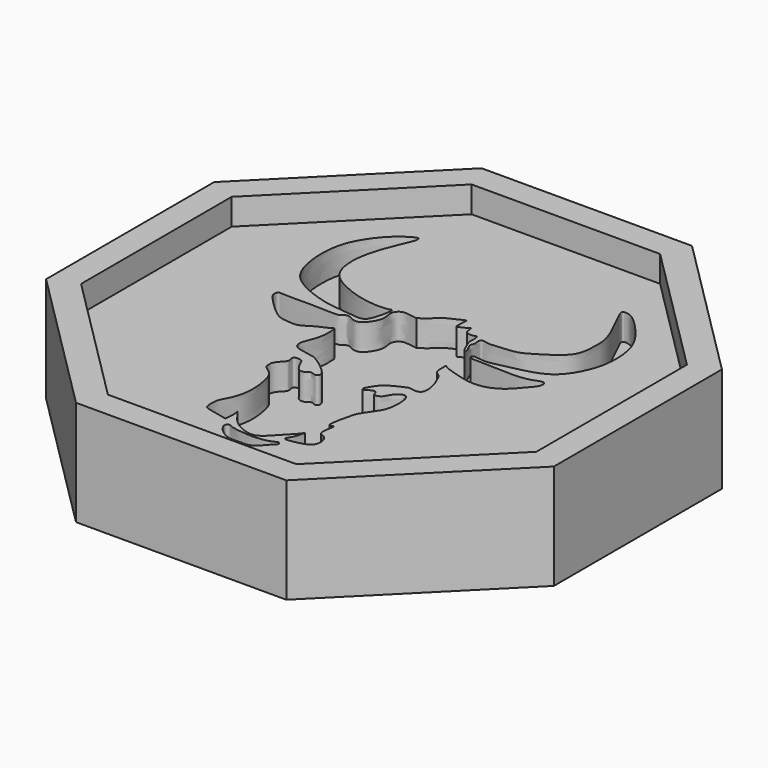
from build123d import *

# Parameters (mm, degrees)
F1_DEPTH = 25.4
F3_DEPTH = 6.35
F5_DEPTH = 6.35


with BuildPart() as f1:
    # F0 (on Top) → F1 (new body)
    with BuildSketch(Plane.XY):
        Polygon((-61.3372846899, 25.3607087968), (-61.3047391097, -25.4392807779), (-25.3607087968, -61.3372846899), (25.4392807779, -61.3047391097), (61.3372846899, -25.3607087968), (61.3047391097, 25.4392807779), (25.3607087968, 61.3372846899), (-25.4392807779, 61.3047391097), align=None)
    extrude(amount=F1_DEPTH)

    # F2 (on face) → F3 (cut)
    with BuildSketch(Plane.XY.offset(25.4)):
        Polygon((-54.9856008905, 22.734521413), (-54.9564255154, -22.8049569991), (-22.734521413, -54.9856008905), (22.8049569991, -54.9564255154), (54.9856008905, -22.734521413), (54.9564255154, 22.8049569991), (22.734521413, 54.9856008905), (-22.8049569991, 54.9564255154), align=None)
    extrude(amount=-F3_DEPTH, mode=Mode.SUBTRACT)

    # F4 (on face) → F5 (cut)
    with BuildSketch(Plane.XY.offset(19.05)):
        with BuildLine():
            add(Edge.make_bspline(
                [(-9.4282692298, -9.2326691374), (-8.4840850857, -9.8260777562), (-6.6516469636, -10.9777435428), (-4.395465984, -13.058877404), (-3.9906127923, -14.1891294159), (-4.8528640078, -15.0271217271), (-6.0855293908, -14.0647696181), (-6.8361021294, -15.0831488918), (-8.4800836888, -15.3844987998), (-9.4607258976, -13.8382234216), (-10.1783295199, -12.39132644), (-10.530585818, -11.4926907531), (-12.7551665659, -11.3984729667), (-12.4444668271, -12.6798354478), (-12.2593299659, -13.6545652797), (-13.6051622467, -14.7620446933), (-14.3409348224, -16.0220239486), (-14.321922051, -16.7704078365), (-14.3138650061, -17.9202545143), (-13.1186034777, -18.6564307431), (-11.4302528187, -20.0472476584), (-10.6225997404, -23.450310294), (-10.1147680829, -28.2741892714), (-11.7415790253, -32.6431531794), (-12.9174382916, -34.1649309464), (-12.9299587644, -37.178912773), (-12.4084055803, -38.2180544166), (-8.2145131464, -38.8077069126), (-6.8308559522, -39.4327185107), (-6.875484581, -38.16030542), (-6.6653450214, -36.0611878603), (-7.371128777, -34.9869994652), (-6.2460552937, -36.5408514888), (-4.4390102983, -39.0530569173), (-1.5015671125, -40.8477543068), (1.7071115917, -41.5564539503), (4.0576467306, -39.4557372162), (6.3424814353, -36.8930641139), (8.1590712868, -35.071811946), (8.5316472223, -34.1183133667), (8.2345836672, -35.2844855117), (7.8610398012, -37.1981099423), (6.2839273245, -38.9874526439), (9.266326691, -38.6346600876), (12.189835357, -37.8890680945), (13.4675883573, -36.1487373368), (12.7198460699, -33.0918695437), (9.930596948, -33.0395399652), (11.7099019289, -28.1494867023), (9.3191604838, -30.1136369501), (10.7720113651, -24.0356712037), (11.150243095, -22.091243294), (13.5772865075, -18.9251935606), (14.8003233954, -16.6011904572), (14.9201164538, -12.1791536076), (13.9622562681, -10.6026640562), (12.7803035011, -10.6938590154), (11.4362744481, -11.9801209333), (10.9312367978, -13.1215024658), (10.2453634757, -14.0686647647), (8.6352191248, -14.3879407439), (8.7073308617, -12.9044764652), (7.5209627677, -12.8396326003), (6.5256616405, -13.580406599), (6.0869976466, -13.9772738505), (5.4570005301, -13.5396377785), (6.3303917881, -11.9377003518), (7.7098741158, -9.8249117821), (11.0587187123, -8.2707570297), (12.4591243746, -7.6294322877), (13.4778087168, -8.1067590986), (15.9277607605, -7.9424041277), (15.2556568662, -3.8663568868), (14.4862990975, -2.3485813704), (13.7665382129, -0.3592892165), (12.2046730698, 0.3939785277), (12.0582121105, 1.6236098482), (12.0255761857, 3.9516208247), (12.4450103136, 3.1027423912), (16.5110699597, 1.8249579504), (21.078106057, 0.7115795625), (26.0638495162, 2.1812531443), (29.2230087502, 5.7843129757), (31.2737116624, 8.2182389542), (31.2278889418, 9.721207294), (30.0857203595, 9.9724642069), (28.472510997, 9.0185412307), (24.5513264234, 8.481216416), (19.6181854574, 8.7905574192), (16.196127468, 8.8653123167), (13.3446161645, 8.723991591), (13.4927937008, 10.2286844933), (16.4508103427, 9.2297816698), (21.1013365186, 10.502293822), (25.9735893436, 11.4472493706), (31.1878588966, 13.4941405465), (34.4638101564, 19.3145293919), (35.6394736154, 24.2110537108), (35.275960363, 31.6512720663), (31.1650423262, 37.2520467873), (28.0533420692, 40.3273925181), (26.4296452657, 41.485700122), (25.4190416812, 41.7070187418), (23.9748134483, 41.8669669932), (24.8551004672, 39.5530018645), (26.5847000727, 36.3840778799), (29.2164222614, 30.8323567036), (28.9476077056, 27.0951272934), (28.9521176027, 21.9651272091), (22.6263582287, 18.0817154192), (19.2763516356, 16.019175046), (15.6410149746, 16.0264947024), (12.6622540075, 15.4454248136), (11.1029074367, 16.2069281425), (10.3960461713, 15.3750494473), (10.8691535509, 13.7673825709), (10.1396442285, 13.0680734148), (11.0848560208, 11.6307606922), (11.6267048162, 9.8553781089), (10.3928447984, 11.2233156131), (9.7992288744, 13.040687065), (9.2598412935, 14.0477513552), (9.579696114, 15.9380770854), (9.0964793415, 16.8614094225), (8.4893205371, 16.2800428745), (6.8331120922, 16.4974540301), (6.4618248238, 16.8524107039), (6.1792797507, 19.1298816215), (5.9113327868, 18.1703634489), (4.4194509507, 17.7211838272), (3.4659487949, 16.9830424479), (3.5619819446, 18.4217518194), (3.5278446131, 19.5784882166), (3.7709848691, 20.6735203119), (2.3441332322, 19.9031610038), (-0.9966306201, 18.4935375741), (-2.3579134542, 16.6290500898), (-3.7437918395, 15.7644089715), (-4.4414699078, 15.3291318566)],
                knots=[0, 0, 0, 0, 0.0093887284, 0.0182213014, 0.0233131476, 0.0280114315, 0.0336124529, 0.0388132789, 0.0448508987, 0.0514661867, 0.0579869925, 0.0628125121, 0.0693776173, 0.0742962539, 0.0792086391, 0.0857519788, 0.0918428882, 0.096206218, 0.1013259694, 0.1071197189, 0.1144428534, 0.1237972835, 0.1352105935, 0.1459420833, 0.1531121172, 0.1615423232, 0.166725975, 0.1771658341, 0.1826563447, 0.1875106221, 0.1953019551, 0.1993991365, 0.2049196268, 0.2142540612, 0.2237371342, 0.2325054811, 0.2411782885, 0.2508781783, 0.2591627147, 0.2628089063, 0.2671087438, 0.2748303973, 0.2810510059, 0.288327223, 0.2974990844, 0.3045293751, 0.3127628534, 0.3198779695, 0.3291877075, 0.3339090751, 0.344899217, 0.3532071168, 0.3628568316, 0.371425535, 0.3819640039, 0.3883300936, 0.3932867711, 0.400116702, 0.405861066, 0.4113515785, 0.4169281938, 0.4220877311, 0.4269420071, 0.4326863712, 0.4363325684, 0.4397829616, 0.4461115588, 0.4544648842, 0.4642024659, 0.4702647327, 0.475518763, 0.4822836579, 0.4917234199, 0.4988296333, 0.5059693952, 0.5122407232, 0.5181217541, 0.5250173913, 0.5279604155, 0.5382313342, 0.5496481242, 0.5608846845, 0.5720957385, 0.5810687061, 0.5864740039, 0.5912025392, 0.597959558, 0.6080841791, 0.6195106459, 0.6293471359, 0.6371175574, 0.6412359933, 0.6492714977, 0.6606297825, 0.672079886, 0.6838871859, 0.6966594462, 0.7081745795, 0.7217890209, 0.7352308346, 0.7458378514, 0.752717581, 0.7579895334, 0.7629390765, 0.7696434146, 0.7798200645, 0.7922806096, 0.8021612881, 0.8130937866, 0.8265476592, 0.8367431308, 0.8462814452, 0.8551661805, 0.8613306134, 0.8658218009, 0.8721503975, 0.8766689416, 0.8833473635, 0.8888875665, 0.8942092607, 0.9015411068, 0.9070011411, 0.9140060991, 0.9183725406, 0.9224140492, 0.928747576, 0.932690837, 0.9394067292, 0.9425824756, 0.9492085016, 0.9537759532, 0.9588705435, 0.9648854784, 0.9691373246, 0.9744837396, 0.9843635518, 0.9921283086, 1, 1, 1, 1], degree=3))
            add(Edge.make_bspline(
                [(-4.4414699078, 15.3291318566), (-4.9068967225, 15.3806827308), (-5.9349556814, 15.4945509834), (-8.2732521375, 15.9847129393), (-9.7667880134, 14.1101988204), (-9.168903392, 12.2312839638), (-9.2484442212, 10.9020733102), (-9.7414335487, 9.5674071396), (-11.3511745418, 7.1567049444), (-13.3918709559, 7.1479473791), (-14.7050111685, 8.1215683651), (-15.5706019088, 7.9667355563), (-16.4311261821, 7.4484853366), (-16.6547257887, 6.9135346109), (-23.4598936578, 7.3918112186), (-29.3448714402, 7.1065466932), (-30.8844644754, 7.3670952023), (-31.5182667154, 7.3409536777), (-31.6997293932, 6.0030194205), (-30.7753763437, 4.6887419911), (-28.3533346738, 2.2006722005), (-24.863507439, -0.8319883365), (-22.4599240989, -0.7963354442), (-20.0140560821, -1.2610430772), (-17.5149487875, 0.8612721058), (-14.8122648285, 1.7088528475), (-14.3728875457, 2.3916052687), (-13.6860658167, 2.380095861), (-13.7189647119, 1.1992723358), (-13.4716632298, -1.5444326183), (-14.9295629485, -5.0303479787), (-15.3564223079, -6.3035501228), (-14.9174930287, -8.246461194), (-12.1365329972, -8.6339063958), (-10.3490742469, -9.0290908364), (-9.4282692298, -9.2326691374)],
                knots=[0, 0, 0, 0, 0.0267259922, 0.0590337618, 0.089461151, 0.1191102068, 0.1435366022, 0.1695820738, 0.2054113012, 0.2347455632, 0.26152597, 0.2813534837, 0.3022021384, 0.3158535767, 0.3709693963, 0.4262535041, 0.4514743551, 0.4660512479, 0.4886049281, 0.5155466217, 0.5566192303, 0.6029135136, 0.6357538083, 0.6683461724, 0.707524857, 0.7435858948, 0.7618014862, 0.7761487209, 0.797006954, 0.8338980252, 0.8758818035, 0.9011714843, 0.9284460361, 0.9631391499, 1, 1, 1, 1], degree=3))
        make_face()
        with BuildLine():
            add(Edge.make_bspline(
                [(-11.9326449931, 8.9084738865), (-11.2962358524, 9.2917720985), (-10.6578160321, 10.9837375729), (-10.1382627959, 13.1078709144), (-9.8502745998, 15.3515303356), (-10.9561982877, 14.5982416136), (-16.5710905244, 14.6323876627), (-23.0669928768, 16.9278992666), (-28.2670840419, 20.4224602133), (-28.9314703073, 28.8125825553), (-25.688544588, 36.8434179775), (-24.4063809769, 39.5778752869), (-24.1592604868, 41.3996816674), (-26.2192121955, 40.5256312351), (-29.9994381949, 37.7589660174), (-34.444888146, 31.2497328496), (-34.9916822779, 24.9324513831), (-34.6879161063, 20.6734445245), (-32.9511608041, 13.932057372), (-25.0337467243, 10.432144423), (-20.2721765186, 9.2808612838), (-15.3825447297, 8.8334678412), (-12.6861217586, 8.4546678701), (-11.9326449931, 8.9084738865)],
                knots=[0, 0, 0, 0, 0.034952122, 0.0714166213, 0.100974403, 0.119845041, 0.1730298163, 0.2348413997, 0.2893685511, 0.3537527211, 0.4214495061, 0.4616313691, 0.4859956187, 0.5136114288, 0.563968818, 0.6283564226, 0.6851056009, 0.73245112, 0.7904650419, 0.8559480448, 0.9075986795, 0.9586184262, 1, 1, 1, 1], degree=3))
        make_face()
        with BuildLine():
            add(Edge.make_bspline(
                [(-0.2690389229, -41.6189283133), (-0.7559459853, -41.5775023038), (-1.9281628917, -41.5464883275), (-2.3116298552, -41.4190567236), (-3.956815349, -41.138282935), (-4.1350406366, -40.9076661362), (-5.041975201, -40.5888659914), (-5.5514031699, -41.4589829371), (-5.0583032619, -42.4082313776), (-4.2408784433, -43.4809876579), (-2.7254620157, -44.541075909), (-1.2224251251, -45.2127540621), (1.3635198147, -44.9904689233), (3.442127916, -45.0751445846), (4.9560675398, -44.0376916587), (6.0685582276, -42.4017388875), (7.6825662355, -41.3073998624), (7.0486044467, -40.3618100068), (6.1474640448, -40.9456318446), (4.5364587935, -41.5027229801), (2.2862829045, -41.754088392), (0.6148836095, -41.75129053), (0.0969062968, -41.6500628999), (-0.2690389229, -41.6189283133)],
                knots=[0, 0, 0, 0, 0.0521070544, 0.0824224864, 0.1334368321, 0.1575458, 0.1938495641, 0.229900884, 0.2708708446, 0.3191172634, 0.3745383858, 0.4271560219, 0.4930882729, 0.5523469847, 0.6058863464, 0.6655393651, 0.7191925586, 0.7525613754, 0.7910566744, 0.8456594271, 0.9087815599, 0.9608378499, 1, 1, 1, 1], degree=3))
        make_face()
    extrude(amount=-F5_DEPTH, mode=Mode.SUBTRACT)


solid = f1.part
